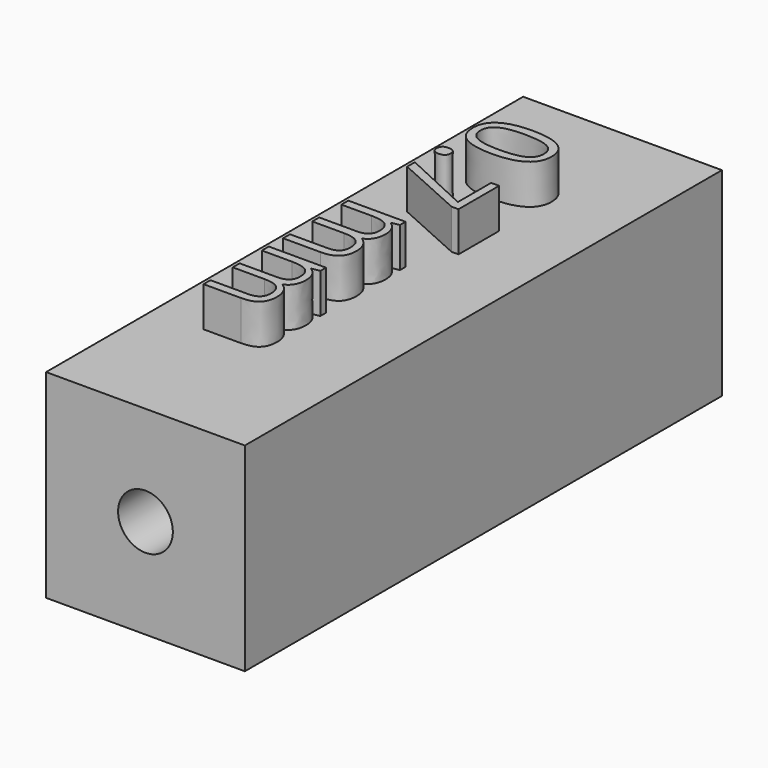
from build123d import *

# Parameters (mm, degrees)
F0_W         = 2.54
F0_H         = 7.62
F1_DEPTH     = 2.54
F2_R         = 0.35000057
F3_DEPTH     = 7.62
F5_TEXT_SIZE = 1.3655100046
F6_DEPTH     = 0.508


# Not quite as in the source:
# - Text() gives the source's letters only with a copy of the font that has no kerning and outlines rounded to 1/6400 em; it was checked with that copy


with BuildPart() as f1:
    # F0 (on Top) → F1 (new body)
    with BuildSketch(Plane.XY):
        with Locations((-1.1584086657, -1.8959715962)):
            Rectangle(F0_W, F0_H)
    extrude(amount=F1_DEPTH)

    # F2 (on face) → F3 (cut)
    with BuildSketch(Plane.XZ.offset(5.7059715962)):
        with Locations((-1.1584086657, 1.27)):
            Circle(F2_R)
    extrude(amount=-F3_DEPTH, mode=Mode.SUBTRACT)

    # F5 (on face) → F6 (join)
    with BuildSketch(Plane.XY.offset(2.54)):
        with Locations(Location((-1.7783786745, 0.7059478658), (0, 0, -90))):
            Text('0.7 mm', F5_TEXT_SIZE, font='Open Sans', text_align=(TextAlign.LEFT, TextAlign.BOTTOM))
    extrude(amount=F6_DEPTH)


solid = f1.part
